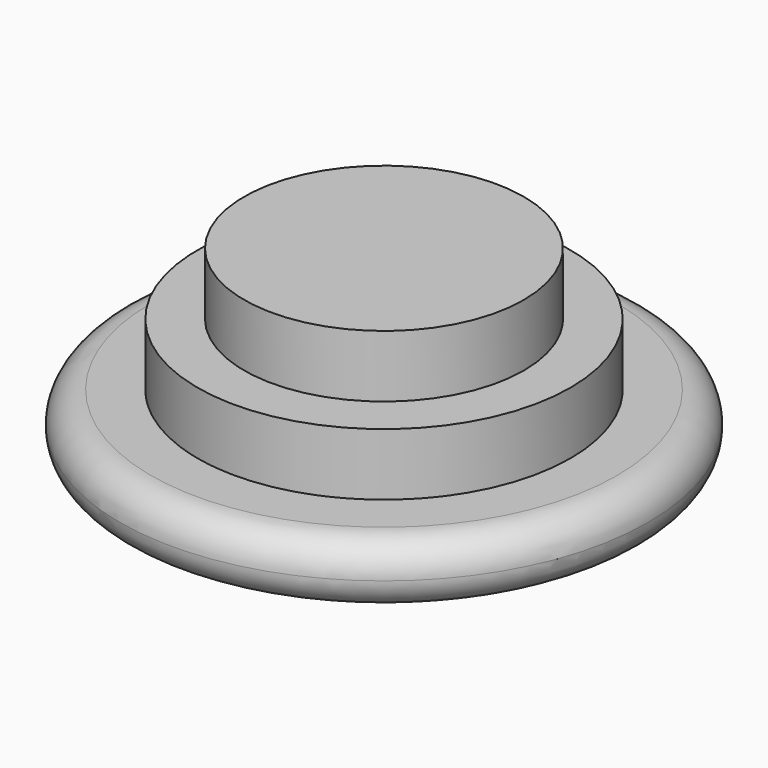
from build123d import *

# Parameters (mm, degrees)
F0_R     = 4.5
F1_DEPTH = 6
F0_R_2   = 6
F2_DEPTH = 4
F0_R_3   = 8.5
F3_DEPTH = 2
F4_R     = 0.99999


# Not quite as in the source:
# - a fillet or chamfer is up to 0.001 mm smaller than in the source, because OpenCascade refuses the exact size


with BuildPart() as f1:
    # F0 (on Top) → F1 (new body)
    with BuildSketch(Plane.XY):
        Circle(F0_R)
    extrude(amount=F1_DEPTH)


with BuildPart() as f2:
    # F0 (on Top) → F2 (new body)
    with BuildSketch(Plane.XY):
        Circle(F0_R_2)
        Circle(F0_R, mode=Mode.SUBTRACT)
    extrude(amount=F2_DEPTH)


with BuildPart() as f3:
    # F0 (on Top) → F3 (new body)
    with BuildSketch(Plane.XY):
        Circle(F0_R_3)
        Circle(F0_R_2, mode=Mode.SUBTRACT)
    extrude(amount=F3_DEPTH)

    # F4 (radius 1 in the source; OpenCascade refuses exactly that, so slightly less here)
    f4_edges = [f3.edges().sort_by_distance(p)[0] for p in [
        (-8.5, 0, 0),
        (-8.5, 0, 2),
    ]]
    fillet(f4_edges, radius=F4_R)


with BuildPart() as f6_tool:
    # F5 (on Front) → F6 (revolve)
    with BuildSketch(Plane.XZ):
        with BuildLine():
            Line((0, 0.7), (0, 0))
            Line((0, 0), (6.5, 0))
            add(Edge.make_bspline(
                [(0, 0.7), (2.7754448838, 0.7950184902), (4.1902936064, 0.3592014255), (6.5, 0)],
                knots=[0, 0, 0, 0, 6.5375836515, 6.5375836515, 6.5375836515, 6.5375836515], degree=3))
        make_face()
    revolve(axis=Axis((0, 0, 0.35), (0, 0, 1)))


with BuildPart() as f1_1:
    add(f1.part)

    # F6: cut by f6_tool
    add(f6_tool.part, mode=Mode.SUBTRACT)


with BuildPart() as f2_1:
    add(f2.part)

    # F6: cut by f6_tool
    add(f6_tool.part, mode=Mode.SUBTRACT)


with BuildPart() as f3_1:
    add(f3.part)

    # F6: cut by f6_tool
    add(f6_tool.part, mode=Mode.SUBTRACT)


solid = Compound([f1_1.part, f2_1.part, f3_1.part])
